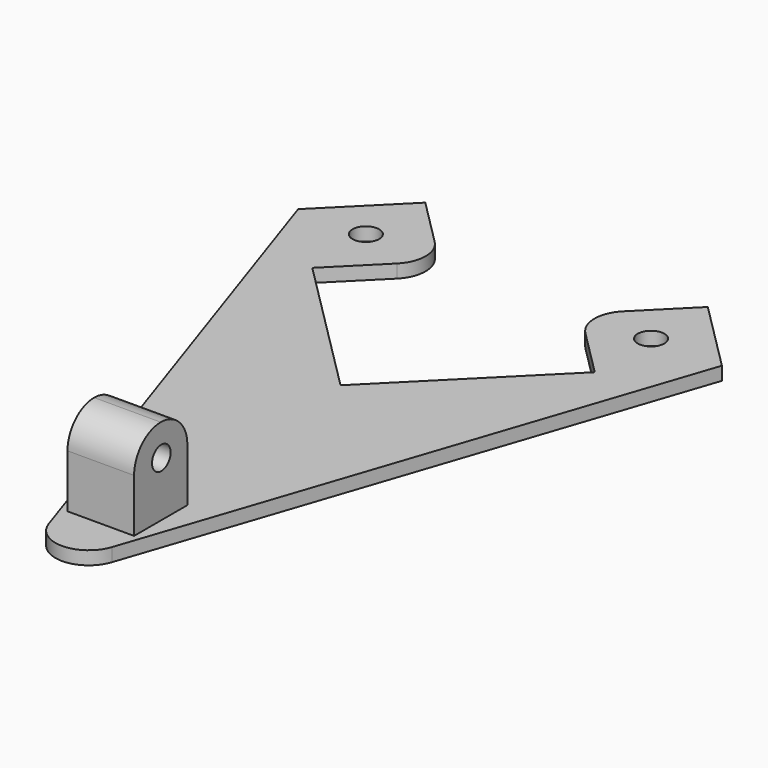
from build123d import *

# Parameters (mm, degrees)
F0_R     = 2
F1_DEPTH = 2
F2_ANGLE = 45
F3_W     = 10
F3_H     = 15
F3_R     = 1.75
F4_DEPTH = 5
F5_R     = 4.99999
F6_R     = 5


# Not quite as in the source:
# - a fillet or chamfer is up to 0.001 mm smaller than in the source, because OpenCascade refuses the exact size


with BuildPart() as f1:
    # F0 (on Top) → F1 (new body)
    with BuildSketch(Plane.XY):
        Polygon((0, 0), (-30, 0), (-30, 15), (-45, 15), (-45, 0), (44.535438389, -44.535438389), (0, 45), (-15, 45), (-15, 30), (0, 30), align=None)
        with Locations((-37.8073789179, 7.1926233359)):
            Circle(F0_R, mode=Mode.SUBTRACT)
        with Locations((-7.745902054, 37.5)):
            Circle(F0_R, mode=Mode.SUBTRACT)
    extrude(amount=F1_DEPTH)


with BuildPart() as f1_1:
    # F2: moved
    add(f1.part.rotate(Axis((0, 0, 1), (0, 0, -1)), F2_ANGLE))

    # F3 (on Right) → F4 (join, symmetric)
    with BuildSketch(Plane.YZ):
        with Locations((-40, 7.5)):
            Rectangle(F3_W, F3_H)
        with Locations((-39.8841314018, 10.2421231568)):
            Circle(F3_R, mode=Mode.SUBTRACT)
    extrude(amount=F4_DEPTH, both=True)

    # F5 (radius 5 in the source; OpenCascade refuses exactly that, so slightly less here)
    f5_edges = [f1_1.edges().sort_by_distance(p)[0] for p in [
        (0, -45, 15),
        (0, -35, 15),
        (10.606602, 31.819805, 1),
        (-10.606602, 31.819805, 1),
    ]]
    fillet(f5_edges, radius=F5_R)

    # F6
    f6_edges = [f1_1.edges().sort_by_distance(p)[0] for p in [
        (0, -62.982621, 1),
    ]]
    fillet(f6_edges, radius=F6_R)


solid = f1_1.part
